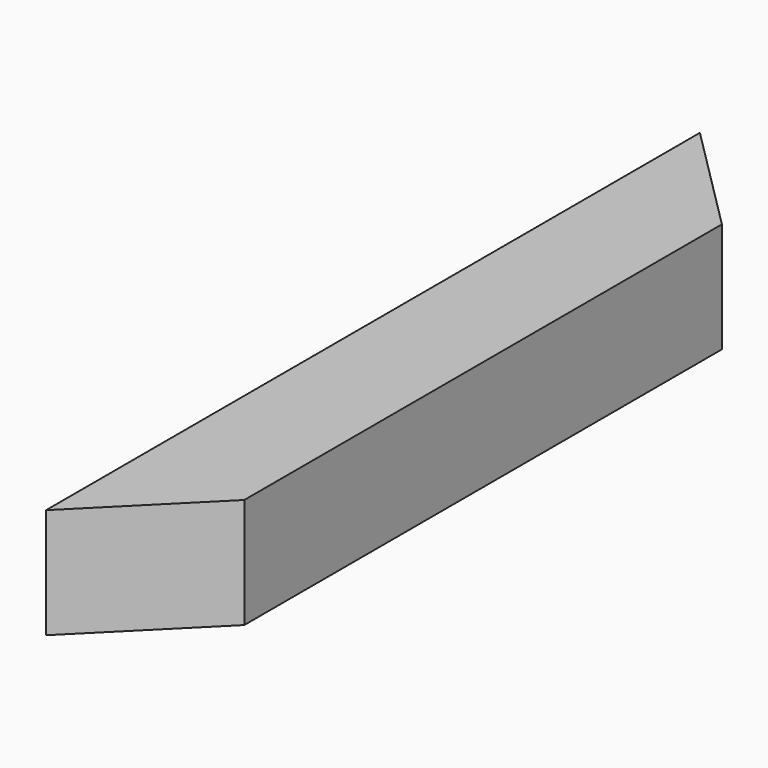
from build123d import *

# Parameters (mm, degrees)
F0_W     = 32.0802
F0_H     = 238.125
F1_DEPTH = 16.0401
F3_DEPTH = 32.0802


# Not quite as in the source:
# - a pattern or mirror of a feature is missing from the dataset's text; its kind, count and spacing are read off the source's solid


with BuildPart() as f1:
    # F0 (on Top) → F1 (new body, symmetric)
    with BuildSketch(Plane.XY):
        Rectangle(F0_W, F0_H)
    extrude(amount=F1_DEPTH, both=True)

    # F2 (on face) → F3 (cut, through all)
    with BuildSketch(Plane.XY.offset(16.0401)):
        Polygon((-16.0401, -119.0625), (16.0401, -119.0625), (16.0401, -86.9823), align=None)
    f3 = extrude(amount=-F3_DEPTH, mode=Mode.SUBTRACT)

    # F3_copies: F3 across plane
    add(f3.mirror(Plane.ZX), mode=Mode.SUBTRACT)


solid = f1.part
